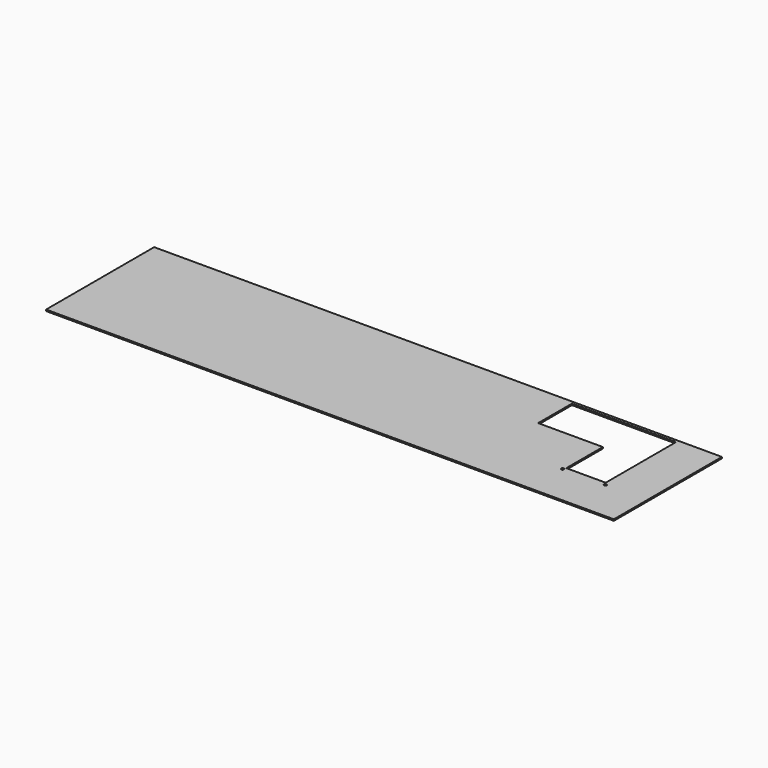
from build123d import *

# Parameters (mm, degrees)
F0_W     = 10248.9
F0_H     = 2438.4
F0_W_2   = 304.8
F0_H_2   = 304.8
F0_R     = 25.4
F1_DEPTH = 25.4


# Not quite as in the source:
# - a feature names something its author has since deleted; it is built from what else it names


with BuildPart() as f1:
    # F0 (on Top) → F1 (new body)
    with BuildSketch(Plane.XY):
        Rectangle(F0_W, F0_H)
        with Locations((-4908.55, -1003.3)):
            Rectangle(F0_W_2, F0_H_2, mode=Mode.SUBTRACT)
        with Locations((1466.85, -1003.3)):
            Rectangle(F0_W_2, F0_H_2, mode=Mode.SUBTRACT)
        with Locations((3600.45, -472.4713563919)):
            Circle(F0_R, mode=Mode.SUBTRACT)
        with Locations((4374.9561309814, -472.4713563919)):
            Circle(F0_R, mode=Mode.SUBTRACT)
        with Locations((-4908.55, 1003.3)):
            Rectangle(F0_W_2, F0_H_2, mode=Mode.SUBTRACT)
        with Locations((2397.383928299, 328.731328249)):
            Circle(F0_R, mode=Mode.SUBTRACT)
        with Locations((3600.45, 328.731328249)):
            Circle(F0_R, mode=Mode.SUBTRACT)
        Polygon((2457.45, 1168.4), (4337.05, 1168.4), (4337.05, -419.1), (3625.85, -419.1), (3625.85, 328.731328249), (3625.85, 406.4), (2457.45, 406.4), align=None, mode=Mode.SUBTRACT)
        with Locations((1466.85, 1003.3)):
            Rectangle(F0_W_2, F0_H_2, mode=Mode.SUBTRACT)
        with Locations((-4908.55, 1003.3)):
            Rectangle(F0_W_2, F0_H_2)
        with Locations((1466.85, 1003.3)):
            Rectangle(F0_W_2, F0_H_2)
        with Locations((1466.85, -1003.3)):
            Rectangle(F0_W_2, F0_H_2)
        with Locations((-4908.55, -1003.3)):
            Rectangle(F0_W_2, F0_H_2)
        with Locations((3600.45, 328.731328249)):
            Circle(F0_R)
        with Locations((2397.383928299, 328.731328249)):
            Circle(F0_R)
    extrude(amount=F1_DEPTH)


solid = f1.part
